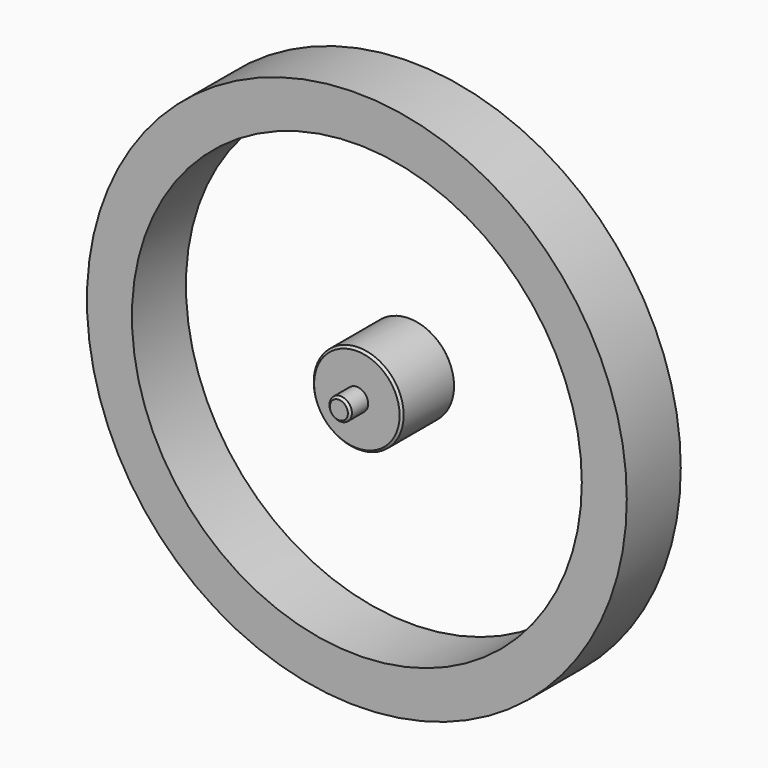
from build123d import *

# Parameters (mm, degrees)
F0_R     = 60
F0_R_2   = 50
F1_DEPTH = 15
F0_R_3   = 10
F2_R     = 2.5
F3_DEPTH = 5
F4_R     = 2.5
F5_DEPTH = 5
F6_SIZE  = 0.5
F7_SIZE  = 0.5
F8_SIZE  = 0.5


# Not quite as in the source:
# - a feature names something its author has since deleted; it is built from what else it names


with BuildPart() as f1:
    # F0 (on Front) → F1 (new body)
    with BuildSketch(Plane.XZ):
        Circle(F0_R)
        Circle(F0_R_2, mode=Mode.SUBTRACT)
    extrude(amount=F1_DEPTH)


with BuildPart() as f1b:
    # F0 (on Front) → F1, piece 2 (new body)
    with BuildSketch(Plane.XZ):
        Circle(F0_R_3)
    extrude(amount=F1_DEPTH)

    # F2 (on face) → F3 (join)
    with BuildSketch(Plane.XZ.offset(15)):
        Circle(F2_R)
    extrude(amount=F3_DEPTH)

    # F4 (on face) → F5 (join)
    with BuildSketch(Plane(origin=(0, 0, 0), x_dir=(-1, 0, 0), z_dir=(0, 1, 0))):
        Circle(F4_R)
    extrude(amount=F5_DEPTH)

    # F6
    f6_edges = [f1b.edges().sort_by_distance(p)[0] for p in [
        (-2.5, -20, 0),
    ]]
    chamfer(f6_edges, length=F6_SIZE)

    # F7
    f7_edges = [f1b.edges().sort_by_distance(p)[0] for p in [
        (10, -7.5, 0),
        (-10, 0, 0),
        (-10, -15, 0),
    ]]
    chamfer(f7_edges, length=F7_SIZE)

    # F8
    f8_edges = [f1b.edges().sort_by_distance(p)[0] for p in [
        (2.5, 5, 0),
    ]]
    chamfer(f8_edges, length=F8_SIZE)


solid = Compound([f1.part, f1b.part])
